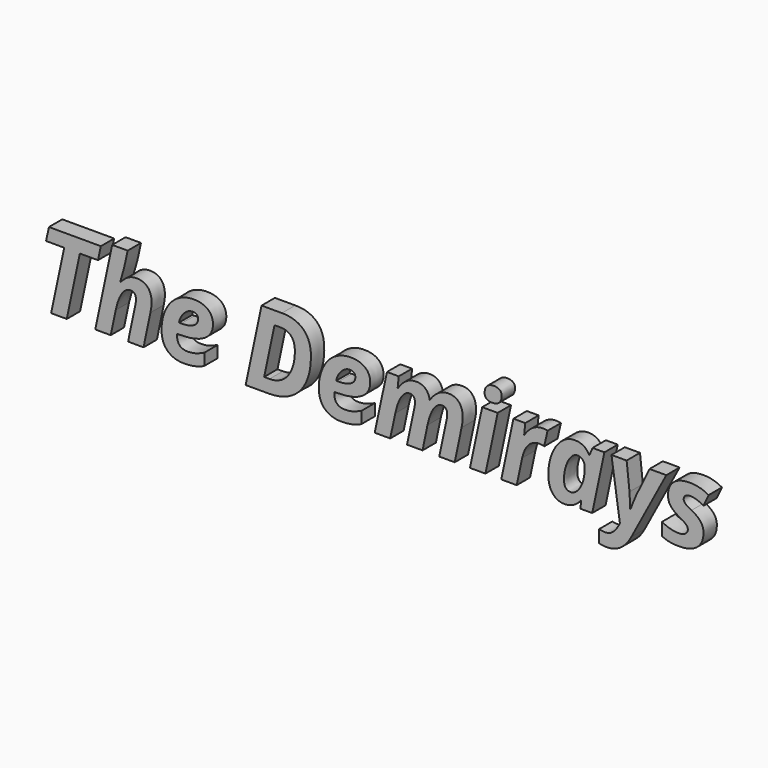
from build123d import *

# Parameters (mm, degrees)
F0_TEXT_SIZE = 160.2013336702
F1_DEPTH     = 25.4


# Not quite as in the source:
# - Text() gives the source's letters only with a copy of the font that has no kerning and outlines rounded to 1/6400 em; it was checked with that copy


with BuildPart() as f1:
    # F0 (on Front) → F1 (new body)
    with BuildSketch(Plane.XZ):
        with Locations((-130.4314732552, -72.1860826015)):
            Text('The Demirays', F0_TEXT_SIZE, font='Open Sans', font_style=FontStyle.BOLDITALIC, text_align=(TextAlign.LEFT, TextAlign.BOTTOM))
    extrude(amount=F1_DEPTH)


solid = f1.part
